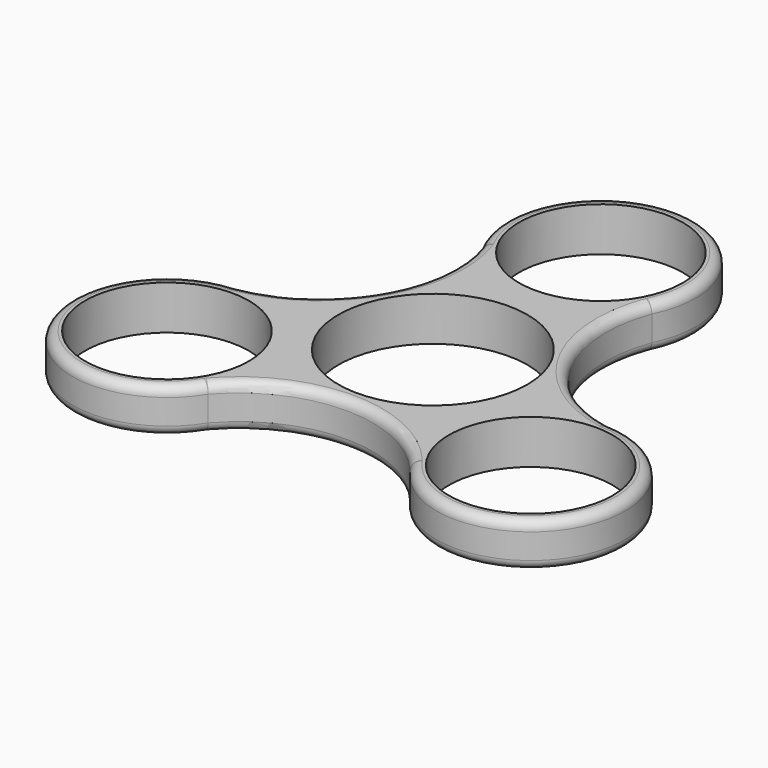
from build123d import *

# Parameters (mm, degrees)
F0_R     = 13
F0_R_2   = 15
F1_DEPTH = 7
F2_R     = 1.5


# Not quite as in the source:
# - a feature names something its author has since deleted; it is built from what else it names


with BuildPart() as f1:
    # F0 (on Top) → F1 (new body)
    with BuildSketch(Plane.XY):
        with BuildLine():
            ThreePointArc((29.2440715105, -1.6706394265), (14.7633799525, 8.8171573496), (13.4280784061, 26.6469436353))
            ThreePointArc((13.4280784061, 26.6469436353), (-0.2737071825, 48.3292581534), (-13.1752195713, 26.1614285514))
            ThreePointArc((-13.1752195713, 26.1614285514), (-15.0175722301, 8.3768834098), (-29.7909693244, -1.6944147939))
            ThreePointArc((-29.7909693244, -1.6944147939), (-41.7175117157, -24.4016664499), (-16.0688519392, -24.4907891249))
            ThreePointArc((-16.0688519392, -24.4907891249), (0.2541922776, -17.1940407594), (16.3628909183, -24.9525288414))
            ThreePointArc((16.3628909183, -24.9525288414), (41.9912188982, -23.9275917035), (29.2440715105, -1.6706394265))
        make_face()
        with Locations((-28.8661470579, -16.6658777744)):
            Circle(F0_R, mode=Mode.SUBTRACT)
        Circle(F0_R_2, mode=Mode.SUBTRACT)
        with Locations((28.8661470579, -16.6658777744)):
            Circle(F0_R, mode=Mode.SUBTRACT)
        with Locations((0, 33.3317555487)):
            Circle(F0_R, mode=Mode.SUBTRACT)
    extrude(amount=F1_DEPTH)

    # F2 (call 1 of 2: OpenCascade refuses the feature's edges together)
    f2_edges = [f1.edges().sort_by_distance(p)[0] for p in [
        (0.254192, -17.194041, 7),
        (-41.717512, -24.401666, 7),
        (-15.017572, 8.376883, 7),
        (14.76338, 8.817157, 7),
        (-0.273707, 48.329258, 7),
        (41.991219, -23.927592, 7),
    ]]
    fillet(f2_edges, radius=F2_R)

    # F2#2 (call 2 of 2)
    f2_2_edges = [f1.edges().sort_by_distance(p)[0] for p in [
        (0.254192, -17.194041, 0),
        (-41.717512, -24.401666, 0),
        (-15.017572, 8.376883, 0),
        (-0.273707, 48.329258, 0),
        (14.76338, 8.817157, 0),
        (41.991219, -23.927592, 0),
    ]]
    fillet(f2_2_edges, radius=F2_R)


solid = f1.part
